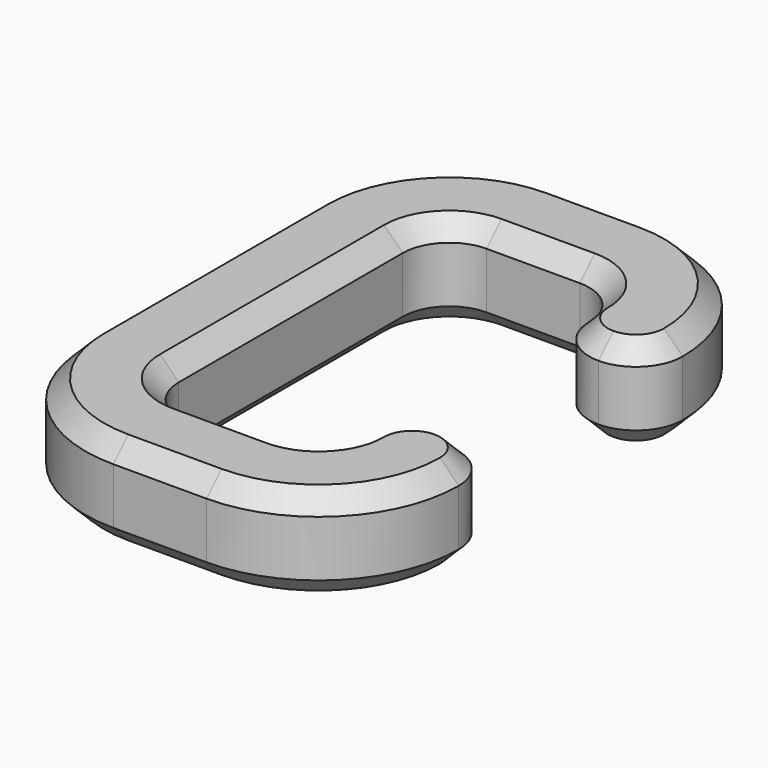
from build123d import *

# Parameters (mm, degrees)
F0_W     = 10
F0_H     = 10
F1_DEPTH = 10
F2_R     = 4.99999
F3_R     = 15
F4_SIZE  = 2


# Not quite as in the source:
# - a fillet or chamfer is up to 0.001 mm smaller than in the source, because OpenCascade refuses the exact size


with BuildPart() as f1:
    # F0 (on Top) → F1 (new body)
    with BuildSketch(Plane.XY):
        Polygon((20, 50), (20, 40), (20, 30), (30, 30), (30, 50), align=None)
        Polygon((-10, 40), (0, 40), (20, 40), (20, 50), (-10, 50), align=None)
        Polygon((0, -10), (0, 0), (0, 40), (-10, 40), (-10, -10), align=None)
        Polygon((20, 0), (0, 0), (0, -10), (30, -10), (30, 0), align=None)
        with Locations((25, 5)):
            Rectangle(F0_W, F0_H)
    extrude(amount=F1_DEPTH)

    # F2 (radius 5 in the source; OpenCascade refuses exactly that, so slightly less here)
    f2_edges = [f1.edges().sort_by_distance(p)[0] for p in [
        (0, 40, 5),
        (20, 30, 5),
        (30, 30, 5),
        (0, 0, 5),
        (20, 10, 5),
        (30, 10, 5),
        (20, 40, 5),
        (20, 0, 5),
    ]]
    fillet(f2_edges, radius=F2_R)

    # F3
    f3_edges = [f1.edges().sort_by_distance(p)[0] for p in [
        (-10, 50, 5),
        (30, 50, 5),
        (30, -10, 5),
        (-10, -10, 5),
    ]]
    fillet(f3_edges, radius=F3_R)

    # F4
    f4_edges = [f1.edges().sort_by_distance(p)[0] for p in [
        (10, 50, 10),
        (10, 50, 0),
    ]]
    chamfer(f4_edges, length=F4_SIZE)


solid = f1.part
